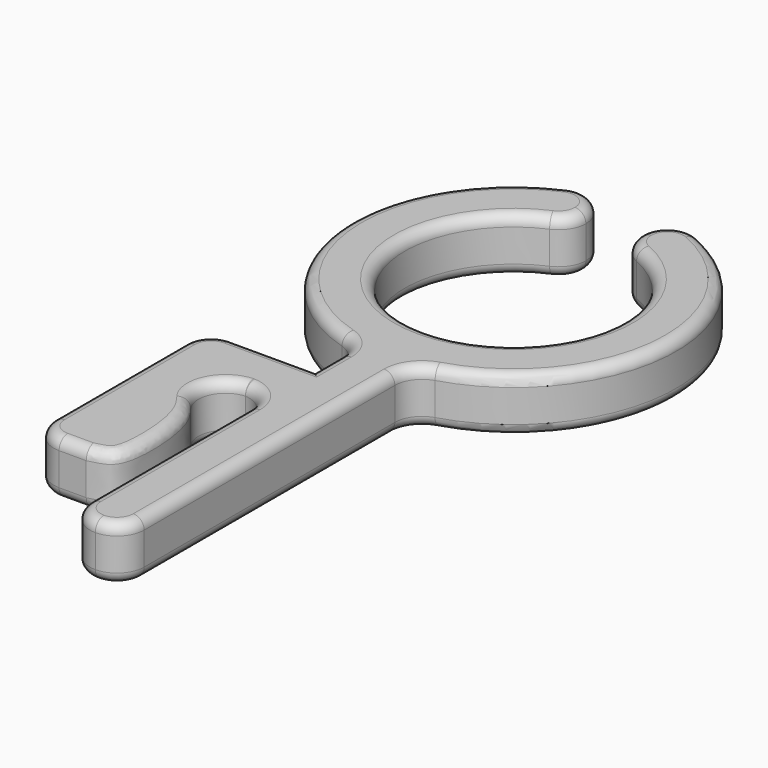
from build123d import *

# Parameters (mm, degrees)
F1_DEPTH    = 3
F2_T1_DEPTH = 3
F2_T3_DEPTH = 3
F3_R        = 0.6
F4_R        = 0.6


# Not quite as in the source:
# - a fillet or chamfer that OpenCascade refuses, or shapes differently, is made with other operations: its cross-section is extruded or revolved along the edge and cut away or added


with BuildPart() as f1:
    # F0 (on Top) → F1 (new body)
    with BuildSketch(Plane.XY):
        with BuildLine():
            ThreePointArc((1.5, 5.8094750193), (0, -6), (-1.5, 5.8094750193))
            Line((-1.5, 5.8094750193), (-1.5, 8.8741196746))
            ThreePointArc((-1.5, 8.8741196746), (-9, 0), (-1.5, -8.8741196746))
            Line((-1.5, -8.8741196746), (-1.5, -11.8741196746))
            Line((-1.5, -11.8741196746), (-1.5, -14.8741196746))
            Line((-1.5, -14.8741196746), (-1.5, -28.8741196746))
            Line((-1.5, -28.8741196746), (1.5, -28.8741196746))
            Line((1.5, -28.8741196746), (1.5, -8.8741196746))
            ThreePointArc((1.5, -8.8741196746), (9, 0), (1.5, 8.8741196746))
            Line((1.5, 8.8741196746), (1.5, 5.8094750193))
        make_face()
        with BuildLine():
            Line((-1.5, -14.8741196746), (-1.5, -11.8741196746))
            Line((-1.5, -11.8741196746), (-7.5, -11.8741196746))
            Line((-7.5, -11.8741196746), (-7.5, -23.8741196746))
            Line((-7.5, -23.8741196746), (-4.5, -23.8741196746))
            add(Edge.make_bspline(
                [(-4.5, -23.8741196746), (-3.9035051329, -23.7296366227), (-2.9994857108, -23.5150595725), (-2.7813660749, -20.9008622396), (-3.2092196663, -17.9917450446), (-4.7523092185, -16.5731869163), (-4.6095842331, -15.4554345531), (-4.5, -14.8741196746)],
                knots=[0, 0, 0, 0, 0.1658918443, 0.3814034098, 0.6267861942, 0.821249495, 1, 1, 1, 1], degree=3))
            Line((-4.5, -14.8741196746), (-1.5, -14.8741196746))
        make_face()
    extrude(amount=F1_DEPTH)

    # F2: fillet of radius 1.5 on 12 edges, made by hand

    # F2_s2 → F2_t1 (join)
    with BuildSketch(Plane.XY):
        with BuildLine():
            ThreePointArc((-4.0176965312, -17.2605849743), (-4.1455161485, -15.6957753482), (-2.8076637744, -14.8741196746))
            Line((-2.8076637744, -14.8741196746), (-2.8076637744, -14.8441196746))
            Line((-2.8076637744, -14.8441196746), (-4.5, -14.8441196746))
            Line((-4.5, -14.8441196746), (-4.529480753, -14.8685622292))
            ThreePointArc((-4.529480753, -14.8685622292), (-4.6180051788, -16.1185168876), (-4.0418971864, -17.2783142803))
            Line((-4.0418971864, -17.2783142803), (-4.0176965312, -17.2605849743))
        make_face()
        with BuildLine():
            ThreePointArc((1.5, -10.0623058987), (1.7973244114, -9.1658844417), (2.5714285714, -8.6248336275))
            Line((2.5714285714, -8.6248336275), (2.5628571429, -8.5960841821))
            ThreePointArc((2.5628571429, -8.5960841821), (2.0327281253, -8.7366421678), (1.495, -8.8445392757))
            Line((1.495, -8.8445392757), (1.47, -8.8741196746))
            Line((1.47, -8.8741196746), (1.47, -10.0623058987))
            Line((1.47, -10.0623058987), (1.5, -10.0623058987))
        make_face()
        with BuildLine():
            ThreePointArc((-3, -14.8741196746), (-1.9393398282, -15.3134595029), (-1.5, -16.3741196746))
            Line((-1.5, -16.3741196746), (-1.47, -16.3741196746))
            Line((-1.47, -16.3741196746), (-1.47, -14.8441196746))
            Line((-1.47, -14.8441196746), (-3, -14.8441196746))
            Line((-3, -14.8441196746), (-3, -14.8741196746))
        make_face()
        with BuildLine():
            ThreePointArc((-2.5714285714, -8.6248336275), (-1.7973244114, -9.1658844417), (-1.5, -10.0623058987))
            Line((-1.5, -10.0623058987), (-1.47, -10.0623058987))
            Line((-1.47, -10.0623058987), (-1.47, -8.8741196746))
            Line((-1.47, -8.8741196746), (-1.495, -8.8445392757))
            ThreePointArc((-1.495, -8.8445392757), (-2.0327281253, -8.7366421678), (-2.5628571429, -8.5960841821))
            Line((-2.5628571429, -8.5960841821), (-2.5714285714, -8.6248336275))
        make_face()
    extrude(amount=F2_T1_DEPTH)

    # F2_s4 → F2_t3 (cut)
    with BuildSketch(Plane.XY):
        with BuildLine():
            ThreePointArc((0, -28.8741196746), (-1.0606601718, -28.4347798464), (-1.5, -27.3741196746))
            Line((-1.5, -27.3741196746), (-1.53, -27.3741196746))
            Line((-1.53, -27.3741196746), (-1.53, -28.9041196746))
            Line((-1.53, -28.9041196746), (0, -28.9041196746))
            Line((0, -28.9041196746), (0, -28.8741196746))
        make_face()
        with BuildLine():
            ThreePointArc((1.5, -27.3741196746), (1.0606601718, -28.4347798464), (0, -28.8741196746))
            Line((0, -28.8741196746), (0, -28.9041196746))
            Line((0, -28.9041196746), (1.53, -28.9041196746))
            Line((1.53, -28.9041196746), (1.53, -27.3741196746))
            Line((1.53, -27.3741196746), (1.5, -27.3741196746))
        make_face()
        with BuildLine():
            ThreePointArc((-6, -23.8741196746), (-7.0606601718, -23.4347798464), (-7.5, -22.3741196746))
            Line((-7.5, -22.3741196746), (-7.53, -22.3741196746))
            Line((-7.53, -22.3741196746), (-7.53, -23.9041196746))
            Line((-7.53, -23.9041196746), (-6, -23.9041196746))
            Line((-6, -23.9041196746), (-6, -23.8741196746))
        make_face()
        with BuildLine():
            ThreePointArc((2.4, 5.4990908339), (1.7450099602, 6.0522797062), (1.5, 6.8738635424))
            Line((1.5, 6.8738635424), (1.47, 6.8738635424))
            Line((1.47, 6.8738635424), (1.47, 5.8094750193))
            Line((1.47, 5.8094750193), (1.4925, 5.7804276442))
            ThreePointArc((1.4925, 5.7804276442), (1.9463849579, 5.6438006339), (2.388, 5.4715953798))
            Line((2.388, 5.4715953798), (2.4, 5.4990908339))
        make_face()
        with BuildLine():
            ThreePointArc((-2.4, 5.4990908339), (-1.7450099602, 6.0522797062), (-1.5, 6.8738635424))
            Line((-1.5, 6.8738635424), (-1.47, 6.8738635424))
            Line((-1.47, 6.8738635424), (-1.47, 5.8094750193))
            Line((-1.47, 5.8094750193), (-1.4925, 5.7804276442))
            ThreePointArc((-1.4925, 5.7804276442), (-1.9463849579, 5.6438006339), (-2.388, 5.4715953798))
            Line((-2.388, 5.4715953798), (-2.4, 5.4990908339))
        make_face()
        with BuildLine():
            ThreePointArc((-1.5, 6.8738635424), (-2.1784161637, 8.1288535822), (-3.6, 8.2486362509))
            Line((-3.6, 8.2486362509), (-3.612, 8.2761317051))
            ThreePointArc((-3.612, 8.2761317051), (-2.5776700263, 8.6542773954), (-1.505, 8.9037000736))
            Line((-1.505, 8.9037000736), (-1.47, 8.8741196746))
            Line((-1.47, 8.8741196746), (-1.47, 6.8738635424))
            Line((-1.47, 6.8738635424), (-1.5, 6.8738635424))
        make_face()
        with BuildLine():
            ThreePointArc((-7.5, -13.3741196746), (-7.0606601718, -12.3134595029), (-6, -11.8741196746))
            Line((-6, -11.8741196746), (-6, -11.8441196746))
            Line((-6, -11.8441196746), (-7.53, -11.8441196746))
            Line((-7.53, -11.8441196746), (-7.53, -13.3741196746))
            Line((-7.53, -13.3741196746), (-7.5, -13.3741196746))
        make_face()
        with BuildLine():
            ThreePointArc((1.5, 6.8738635424), (2.1784161637, 8.1288535822), (3.6, 8.2486362509))
            Line((3.6, 8.2486362509), (3.612, 8.2761317051))
            ThreePointArc((3.612, 8.2761317051), (2.5776700263, 8.6542773954), (1.505, 8.9037000736))
            Line((1.505, 8.9037000736), (1.47, 8.8741196746))
            Line((1.47, 8.8741196746), (1.47, 6.8738635424))
            Line((1.47, 6.8738635424), (1.5, 6.8738635424))
        make_face()
    extrude(amount=F2_T3_DEPTH, mode=Mode.SUBTRACT)

    # F3
    f3_edges = [f1.edges().sort_by_distance(p)[0] for p in [
        (2.178416, 8.128854, 3),
        (8.983325, -0.547605, 3),
        (1.797324, -9.165884, 3),
        (1.5, -18.718213, 3),
        (1.06066, -28.43478, 3),
        (-1.06066, -28.43478, 3),
        (-1.5, -21.87412, 3),
        (-1.905867, -15.348023, 3),
        (-4.166584, -15.739033, 3),
        (-2.896337, -20.883795, 3),
        (-5.25, -23.87412, 3),
        (-7.06066, -23.43478, 3),
        (-7.5, -17.87412, 3),
        (-7.06066, -12.31346, 3),
        (-3.75, -11.87412, 3),
        (-1.5, -10.968213, 3),
        (-1.797324, -9.165884, 3),
        (-8.983325, -0.547605, 3),
        (-2.178416, 8.128854, 3),
        (-1.74501, 6.05228, 3),
        (0, -6, 3),
        (1.74501, 6.05228, 3),
    ]]
    fillet(f3_edges, radius=F3_R)

    # F4
    f4_edges = [f1.edges().sort_by_distance(p)[0] for p in [
        (2.178416, 8.128854, 0),
        (8.983325, -0.547605, 0),
        (1.797324, -9.165884, 0),
        (1.5, -18.718213, 0),
        (1.06066, -28.43478, 0),
        (-1.06066, -28.43478, 0),
        (-1.5, -21.87412, 0),
        (-1.905867, -15.348023, 0),
        (-4.166584, -15.739033, 0),
        (-2.896337, -20.883795, 0),
        (-5.25, -23.87412, 0),
        (-7.06066, -23.43478, 0),
        (-7.5, -17.87412, 0),
        (-7.06066, -12.31346, 0),
        (-3.75, -11.87412, 0),
        (-1.5, -10.968213, 0),
        (-1.797324, -9.165884, 0),
        (-8.983325, -0.547605, 0),
        (-2.178416, 8.128854, 0),
        (-1.74501, 6.05228, 0),
        (0, -6, 0),
        (1.74501, 6.05228, 0),
    ]]
    fillet(f4_edges, radius=F4_R)


solid = f1.part
